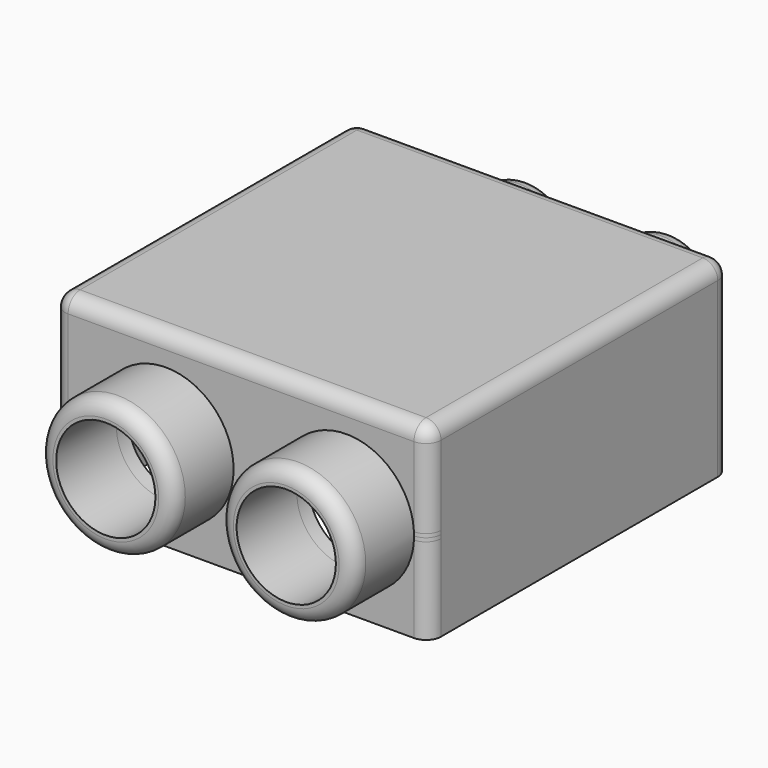
from build123d import *

# Parameters (mm, degrees)
F0_W     = 25
F0_H     = 12.5
F0_R     = 3.25
F0_R_2   = 2.5
F1_DEPTH = 25
F2_T     = -1
F3_DEPTH = 10
F4_DEPTH = 5
F5_R     = 3.3
F6_DEPTH = 10
F5_R_2   = 4.5
F7_DEPTH = 5
F8_R     = 1


# Not quite as in the source:
# - a fillet or chamfer that OpenCascade refuses, or shapes differently, is made with other operations: its cross-section is extruded or revolved along the edge and cut away or added


with BuildPart() as f1:
    # F0 (on Front) → F1 (new body)
    with BuildSketch(Plane.XZ):
        with Locations((1.7170939115, 9.0107331052)):
            Rectangle(F0_W, F0_H)
        with Locations((-3.0594504727, 9.0107331052)):
            Circle(F0_R, mode=Mode.SUBTRACT)
        with Locations((6.4404988661, 9.0417582542)):
            Circle(F0_R, mode=Mode.SUBTRACT)
        with Locations((-3.0594504727, 9.0107331052)):
            Circle(F0_R)
        with Locations((-3.0594504727, 9.0107331052)):
            Circle(F0_R_2, mode=Mode.SUBTRACT)
        with Locations((6.4404988661, 9.0417582542)):
            Circle(F0_R)
        with Locations((6.4404988661, 9.0417582542)):
            Circle(F0_R_2, mode=Mode.SUBTRACT)
        with Locations((-3.0594504727, 9.0107331052)):
            Circle(F0_R_2)
        with Locations((6.4404988661, 9.0417582542)):
            Circle(F0_R_2)
    extrude(amount=F1_DEPTH)

    # F2
    f2_openings = [f1.faces().sort_by_distance(p)[0] for p in [
        (1.717094, -12.5, 2.760733),
    ]]
    offset(amount=F2_T, openings=f2_openings)

    # F0 (on Front) → F3 (cut)
    with BuildSketch(Plane.XZ):
        with Locations((6.4404988661, 9.0417582542)):
            Circle(F0_R_2)
        with Locations((-3.0594504727, 9.0107331052)):
            Circle(F0_R_2)
    extrude(amount=F3_DEPTH, mode=Mode.SUBTRACT)

    # F0 (on Front) → F4 (join)
    with BuildSketch(Plane.XZ):
        with Locations((-3.0594504727, 9.0107331052)):
            Circle(F0_R)
        with Locations((-3.0594504727, 9.0107331052)):
            Circle(F0_R_2, mode=Mode.SUBTRACT)
        with Locations((6.4404988661, 9.0417582542)):
            Circle(F0_R)
        with Locations((6.4404988661, 9.0417582542)):
            Circle(F0_R_2, mode=Mode.SUBTRACT)
    extrude(amount=-F4_DEPTH)

    # F5 (on face) → F6 (cut)
    with BuildSketch(Plane.XZ.offset(25)):
        with Locations((-3.2763871515, 8.743028397)):
            Circle(F5_R)
        with Locations((8.7236128485, 8.743028397)):
            Circle(F5_R)
    extrude(amount=-F6_DEPTH, mode=Mode.SUBTRACT)

    # F5 (on face) → F7 (join)
    with BuildSketch(Plane.XZ.offset(25)):
        with Locations((-3.2763871515, 8.743028397)):
            Circle(F5_R_2)
        with Locations((-3.2763871515, 8.743028397)):
            Circle(F5_R, mode=Mode.SUBTRACT)
        with Locations((8.7236128485, 8.743028397)):
            Circle(F5_R_2)
        with Locations((8.7236128485, 8.743028397)):
            Circle(F5_R, mode=Mode.SUBTRACT)
    extrude(amount=F7_DEPTH)

    # F8
    f8_edges = [f1.edges().sort_by_distance(p)[0] for p in [
        (14.217094, -25, 9.010733),
        (14.217094, -12.5, 15.260733),
        (1.717094, -25, 15.260733),
        (-10.782906, -25, 9.010733),
        (14.217094, 0, 9.010733),
        (1.717094, 0, 15.260733),
        (-10.782906, 0, 9.010733),
        (-10.782906, -12.5, 15.260733),
    ]]
    fillet(f8_edges, radius=F8_R)

    # F9: fillet of radius 1 on 4 edges, made by hand

    # F9_s1 → F9_t2 (revolve, cut)
    with BuildSketch(Plane.XY.offset(9.0417582542)):
        with BuildLine():
            ThreePointArc((9.6906488661, 4.0318703599), (9.4811826994, 4.6442887287), (8.9405363493, 5.0001452412))
            Line((8.9405363493, 5.0001452412), (8.9455340989, 5.0195107389))
            ThreePointArc((8.9455340989, 5.0195107389), (9.3155176077, 5.02), (9.6904988661, 5.02))
            Line((9.6904988661, 5.02), (9.7104988661, 5))
            ThreePointArc((9.7104988661, 5), (9.7104988661, 4.51593518), (9.7106488661, 4.0318703599))
            Line((9.7106488661, 4.0318703599), (9.6906488661, 4.0318703599))
        make_face()
    revolve(axis=Axis((6.4404988661, 5, 9.0417582542), (0, -1, 0)), mode=Mode.SUBTRACT)

    # F9_s3 → F9_t4 (revolve, cut)
    with BuildSketch(Plane.XY.offset(9.0107331052)):
        with BuildLine():
            ThreePointArc((0.1906995273, 4.0318703599), (-0.0187666394, 4.6442887287), (-0.5594129896, 5.0001452412))
            Line((-0.5594129896, 5.0001452412), (-0.5544152399, 5.0195107389))
            ThreePointArc((-0.5544152399, 5.0195107389), (-0.1844317311, 5.02), (0.1905495273, 5.02))
            Line((0.1905495273, 5.02), (0.2105495273, 5))
            ThreePointArc((0.2105495273, 5), (0.2105495273, 4.51593518), (0.2106995273, 4.0318703599))
            Line((0.2106995273, 4.0318703599), (0.1906995273, 4.0318703599))
        make_face()
    revolve(axis=Axis((-3.0594504727, 5, 9.0107331052), (0, -1, 0)), mode=Mode.SUBTRACT)

    # F9_s5 → F9_t6 (revolve, cut)
    with BuildSketch(Plane.XY.offset(8.743028397)):
        with BuildLine():
            ThreePointArc((1.2237628485, -29.00015), (0.9308696297, -29.7072567812), (0.2237628485, -30.00015))
            Line((0.2237628485, -30.00015), (0.2237628485, -30.02015))
            ThreePointArc((0.2237628485, -30.02015), (0.7236878485, -30.02), (1.2236128485, -30.02))
            Line((1.2236128485, -30.02), (1.2436128485, -30))
            ThreePointArc((1.2436128485, -30), (1.2436128485, -29.500075), (1.2437628485, -29.00015))
            Line((1.2437628485, -29.00015), (1.2237628485, -29.00015))
        make_face()
    revolve(axis=Axis((-3.2763871515, -30, 8.743028397), (0, -1, 0)), mode=Mode.SUBTRACT)

    # F9_s7 → F9_t8 (revolve, cut)
    with BuildSketch(Plane.XY.offset(8.743028397)):
        with BuildLine():
            ThreePointArc((13.2237628485, -29.00015), (12.9308696297, -29.7072567812), (12.2237628485, -30.00015))
            Line((12.2237628485, -30.00015), (12.2237628485, -30.02015))
            ThreePointArc((12.2237628485, -30.02015), (12.7236878485, -30.02), (13.2236128485, -30.02))
            Line((13.2236128485, -30.02), (13.2436128485, -30))
            ThreePointArc((13.2436128485, -30), (13.2436128485, -29.500075), (13.2437628485, -29.00015))
            Line((13.2437628485, -29.00015), (13.2237628485, -29.00015))
        make_face()
    revolve(axis=Axis((8.7236128485, -30, 8.743028397), (0, -1, 0)), mode=Mode.SUBTRACT)


solid = f1.part
